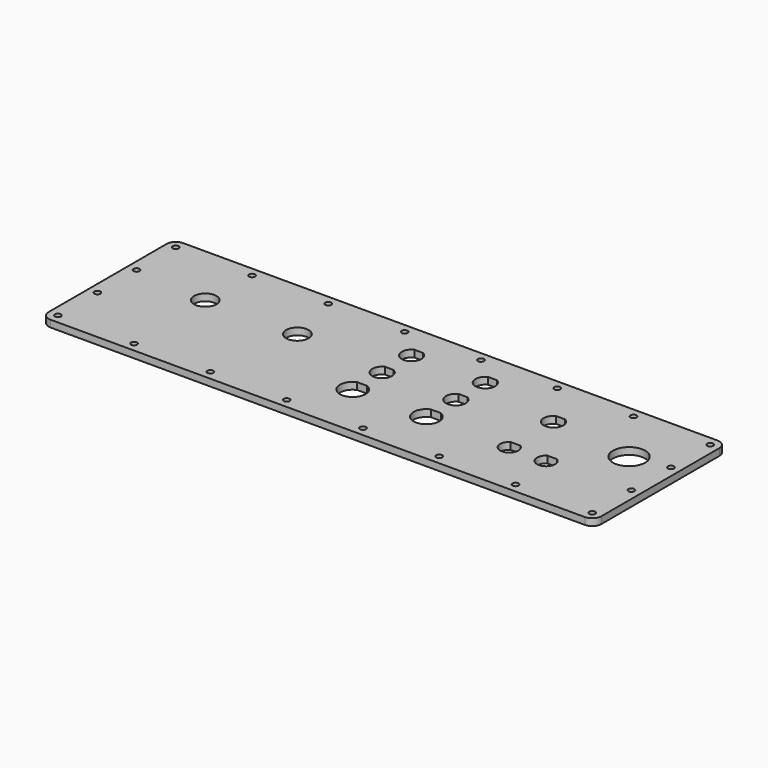
from build123d import *

# Parameters (mm, degrees)
F0_R     = 7.747
F0_R_2   = 11.15
F1_DEPTH = 4.7625
F3_D     = 4.1656


# Not quite as in the source:
# - a feature names something its author has since deleted; it is built from what else it names


with BuildPart() as f1:
    # F0 (on Top) → F1 (new body)
    with BuildSketch(Plane.XY):
        with BuildLine():
            Line((219.054815799, 72.2457910836), (-149.245184201, 72.2457910836))
            ThreePointArc((-149.245184201, 72.2457910836), (-153.7353122615, 70.3859191441), (-155.595184201, 65.8957910836))
            Line((-155.595184201, 65.8957910836), (-155.595184201, -35.7042089164))
            ThreePointArc((-155.595184201, -35.7042089164), (-153.7353122615, -40.194336977), (-149.245184201, -42.0542089164))
            Line((-149.245184201, -42.0542089164), (219.054815799, -42.0542089164))
            ThreePointArc((219.054815799, -42.0542089164), (223.5449438595, -40.194336977), (225.404815799, -35.7042089164))
            Line((225.404815799, -35.7042089164), (225.404815799, 65.8957910836))
            ThreePointArc((225.404815799, 65.8957910836), (223.5449438595, 70.3859191441), (219.054815799, 72.2457910836))
        make_face()
        with BuildLine():
            ThreePointArc((31.9875588712, 4.1757910836), (35.9092220501, 0.923632173), (37.379815799, -3.9542089164))
            ThreePointArc((37.379815799, -3.9542089164), (23.6769747096, -11.3086151675), (25.1220727268, 4.1757910836))
            ThreePointArc((25.1220727268, 4.1757910836), (28.554815799, 4.8707910836), (31.9875588712, 4.1757910836))
        make_face(mode=Mode.SUBTRACT)
        with BuildLine():
            ThreePointArc((82.7875588712, 4.1757910836), (86.7092220501, 0.923632173), (88.179815799, -3.9542089164))
            ThreePointArc((88.179815799, -3.9542089164), (74.4769747096, -11.3086151675), (75.9220727268, 4.1757910836))
            ThreePointArc((75.9220727268, 4.1757910836), (79.354815799, 4.8707910836), (82.7875588712, 4.1757910836))
        make_face(mode=Mode.SUBTRACT)
        with BuildLine():
            ThreePointArc((139.8959807906, 1.2957910836), (141.9937720385, -0.965252677), (142.754815799, -3.9542089164))
            ThreePointArc((142.754815799, -3.9542089164), (133.5158595595, -9.4431651559), (133.1136508074, 1.2957910836))
            ThreePointArc((133.1136508074, 1.2957910836), (136.504815799, 2.2957910836), (139.8959807906, 1.2957910836))
        make_face(mode=Mode.SUBTRACT)
        with BuildLine():
            ThreePointArc((165.2959807906, 1.2957910836), (167.3937720385, -0.965252677), (168.154815799, -3.9542089164))
            ThreePointArc((168.154815799, -3.9542089164), (158.9158595595, -9.4431651559), (158.5136508074, 1.2957910836))
            ThreePointArc((158.5136508074, 1.2957910836), (161.904815799, 2.2957910836), (165.2959807906, 1.2957910836))
        make_face(mode=Mode.SUBTRACT)
        with Locations((-98.445184201, 27.7957910836)):
            Circle(F0_R, mode=Mode.SUBTRACT)
        with Locations((-34.945184201, 27.7957910836)):
            Circle(F0_R, mode=Mode.SUBTRACT)
        with BuildLine():
            ThreePointArc((31.5598116393, 27.5457910836), (34.3286348, 25.0378676617), (35.354815799, 21.4457910836))
            ThreePointArc((35.354815799, 21.4457910836), (24.9627392209, 15.6719720825), (25.5498199587, 27.5457910836))
            ThreePointArc((25.5498199587, 27.5457910836), (28.554815799, 28.2457910836), (31.5598116393, 27.5457910836))
        make_face(mode=Mode.SUBTRACT)
        with BuildLine():
            ThreePointArc((31.5598116393, 52.9457910836), (34.3286348, 50.4378676617), (35.354815799, 46.8457910836))
            ThreePointArc((35.354815799, 46.8457910836), (24.9627392209, 41.0719720825), (25.5498199587, 52.9457910836))
            ThreePointArc((25.5498199587, 52.9457910836), (28.554815799, 53.6457910836), (31.5598116393, 52.9457910836))
        make_face(mode=Mode.SUBTRACT)
        with BuildLine():
            ThreePointArc((82.3533070463, 27.5489910836), (85.1267193187, 25.0409447325), (86.154815799, 21.4457910836))
            ThreePointArc((86.154815799, 21.4457910836), (75.7596621501, 15.6738875639), (76.3563245517, 27.5489910836))
            ThreePointArc((76.3563245517, 27.5489910836), (79.354815799, 28.2457910836), (82.3533070463, 27.5489910836))
        make_face(mode=Mode.SUBTRACT)
        with Locations((193.654815799, 27.7957910836)):
            Circle(F0_R_2, mode=Mode.SUBTRACT)
        with BuildLine():
            ThreePointArc((139.5098116393, 40.2457910836), (142.2786348, 37.7378676617), (143.304815799, 34.1457910836))
            ThreePointArc((143.304815799, 34.1457910836), (132.9127392209, 28.3719720825), (133.4998199587, 40.2457910836))
            ThreePointArc((133.4998199587, 40.2457910836), (136.504815799, 40.9457910836), (139.5098116393, 40.2457910836))
        make_face(mode=Mode.SUBTRACT)
        with BuildLine():
            ThreePointArc((82.3533070463, 52.9489910836), (85.1267193187, 50.4409447325), (86.154815799, 46.8457910836))
            ThreePointArc((86.154815799, 46.8457910836), (75.7596621501, 41.0738875639), (76.3563245517, 52.9489910836))
            ThreePointArc((76.3563245517, 52.9489910836), (79.354815799, 53.6457910836), (82.3533070463, 52.9489910836))
        make_face(mode=Mode.SUBTRACT)
        with BuildLine():
            Line((158.5136508074, 1.2957910836), (165.2959807906, 1.2957910836))
            ThreePointArc((165.2959807906, 1.2957910836), (161.904815799, 2.2957910836), (158.5136508074, 1.2957910836))
        make_face()
        with BuildLine():
            Line((133.1136508074, 1.2957910836), (139.8959807906, 1.2957910836))
            ThreePointArc((139.8959807906, 1.2957910836), (136.504815799, 2.2957910836), (133.1136508074, 1.2957910836))
        make_face()
        with BuildLine():
            Line((25.1220727268, 4.1757910836), (31.9875588712, 4.1757910836))
            ThreePointArc((31.9875588712, 4.1757910836), (28.554815799, 4.8707910836), (25.1220727268, 4.1757910836))
        make_face()
        with BuildLine():
            Line((75.9220727268, 4.1757910836), (82.7875588712, 4.1757910836))
            ThreePointArc((82.7875588712, 4.1757910836), (79.354815799, 4.8707910836), (75.9220727268, 4.1757910836))
        make_face()
        with BuildLine():
            Line((133.4998199587, 40.2457910836), (139.5098116393, 40.2457910836))
            ThreePointArc((139.5098116393, 40.2457910836), (136.504815799, 40.9457910836), (133.4998199587, 40.2457910836))
        make_face()
        with BuildLine():
            Line((25.5498199587, 52.9457910836), (31.5598116393, 52.9457910836))
            ThreePointArc((31.5598116393, 52.9457910836), (28.554815799, 53.6457910836), (25.5498199587, 52.9457910836))
        make_face()
        with BuildLine():
            Line((76.3563245517, 52.9489910836), (82.3533070463, 52.9489910836))
            ThreePointArc((82.3533070463, 52.9489910836), (79.354815799, 53.6457910836), (76.3563245517, 52.9489910836))
        make_face()
        with BuildLine():
            Line((76.3563245517, 27.5489910836), (82.3533070463, 27.5489910836))
            ThreePointArc((82.3533070463, 27.5489910836), (79.354815799, 28.2457910836), (76.3563245517, 27.5489910836))
        make_face()
        with BuildLine():
            Line((25.5498199587, 27.5457910836), (31.5598116393, 27.5457910836))
            ThreePointArc((31.5598116393, 27.5457910836), (28.554815799, 28.2457910836), (25.5498199587, 27.5457910836))
        make_face()
    extrude(amount=F1_DEPTH)

    # F3 (through all)
    with Locations(Plane.XY.offset(4.7625)):
        with Locations((-149.245184201, 65.8957910836), (-149.245184201, -35.7042089164), (219.054815799, 65.8957910836), (219.054815799, -35.7042089164), (-96.667184201, 65.8957910836), (113.644815799, 65.8957910836), (61.066815799, 65.8957910836), (166.222815799, 65.8957910836), (8.488815799, 65.8957910836), (-44.089184201, 65.8957910836), (-149.245184201, -1.6682089164), (-149.245184201, 32.1137910836), (61.066815799, -35.7042089164), (166.222815799, -35.7042089164), (-96.667184201, -35.7042089164), (-44.089184201, -35.7042089164), (113.644815799, -35.7042089164), (8.488815799, -35.7042089164), (219.054815799, -1.9222089164), (219.054815799, 32.1137910836)):
            Hole(F3_D / 2)


solid = f1.part
